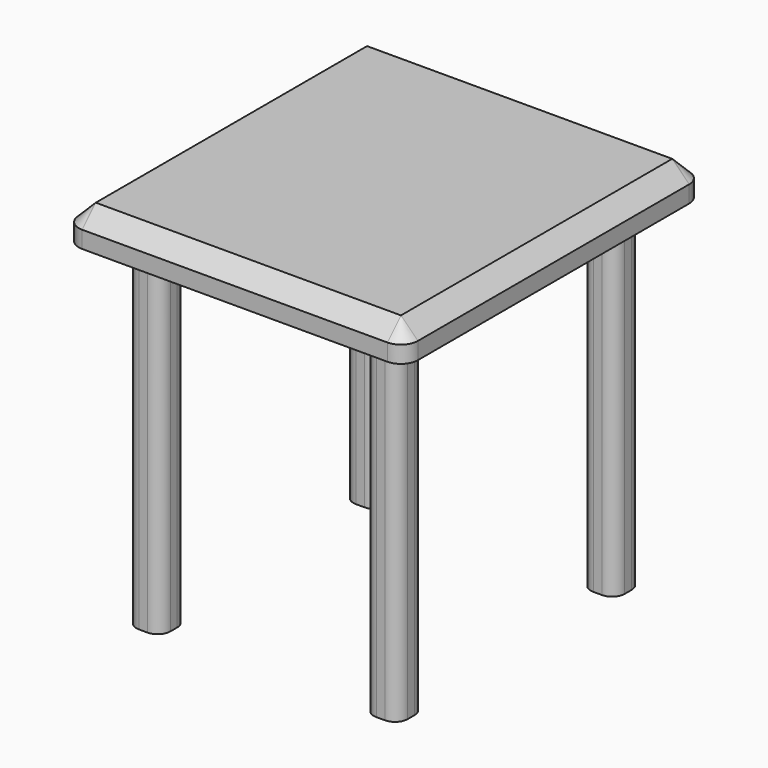
from build123d import *

# Parameters (mm, degrees)
F1_DEPTH = 40
F3_DEPTH = 400
F4_SIZE  = 19.99999


# Not quite as in the source:
# - a fillet or chamfer is up to 0.001 mm smaller than in the source, because OpenCascade refuses the exact size


with BuildPart() as f1:
    # F0 (on Top) → F1 (new body)
    with BuildSketch(Plane.XY):
        with BuildLine():
            Line((182.8182994574, 235.7496355578), (-177.1817005426, 235.7496355578))
            ThreePointArc((-177.1817005426, 235.7496355578), (-191.3238361663, 229.8917711815), (-197.1817005426, 215.7496355578))
            Line((-197.1817005426, 215.7496355578), (-197.1817005426, -184.2503644422))
            ThreePointArc((-197.1817005426, -184.2503644422), (-191.3238361663, -198.3925000659), (-177.1817005426, -204.2503644422))
            Line((-177.1817005426, -204.2503644422), (182.8182994574, -204.2503644422))
            ThreePointArc((182.8182994574, -204.2503644422), (196.9604350812, -198.3925000659), (202.8182994574, -184.2503644422))
            Line((202.8182994574, -184.2503644422), (202.8182994574, 215.7496355578))
            ThreePointArc((202.8182994574, 215.7496355578), (196.9604350812, 229.8917711815), (182.8182994574, 235.7496355578))
        make_face()
    extrude(amount=F1_DEPTH)

    # F2 (on face) → F3 (join)
    with BuildSketch(Plane(origin=(0, 0, 0), x_dir=(1, 0, 0), z_dir=(0, 0, -1))):
        with BuildLine():
            Line((-155.6743295648, -195.7496355578), (-132.1817005426, -195.7496355578))
            ThreePointArc((-132.1817005426, -195.7496355578), (-121.5750988248, -191.3562372756), (-117.1817005426, -180.7496355578))
            Line((-117.1817005426, -180.7496355578), (-117.1817005426, -170.7496355578))
            ThreePointArc((-117.1817005426, -170.7496355578), (-121.5750988248, -160.14303384), (-132.1817005426, -155.7496355578))
            Line((-132.1817005426, -155.7496355578), (-142.1817005426, -155.7496355578))
            ThreePointArc((-142.1817005426, -155.7496355578), (-152.7883022604, -160.14303384), (-157.1817005426, -170.7496355578))
            Line((-157.1817005426, -170.7496355578), (-157.1817005426, -194.2422645801))
            ThreePointArc((-157.1817005426, -194.2422645801), (-156.740201805, -195.3081368202), (-155.6743295648, -195.7496355578))
        make_face()
        with BuildLine():
            Line((124.3256704352, -195.7496355578), (147.8182994574, -195.7496355578))
            ThreePointArc((147.8182994574, -195.7496355578), (158.4249011752, -191.3562372756), (162.8182994574, -180.7496355578))
            Line((162.8182994574, -180.7496355578), (162.8182994574, -170.7496355578))
            ThreePointArc((162.8182994574, -170.7496355578), (158.4249011752, -160.14303384), (147.8182994574, -155.7496355578))
            Line((147.8182994574, -155.7496355578), (137.8182994574, -155.7496355578))
            ThreePointArc((137.8182994574, -155.7496355578), (127.2116977396, -160.14303384), (122.8182994574, -170.7496355578))
            Line((122.8182994574, -170.7496355578), (122.8182994574, -194.2422645801))
            ThreePointArc((122.8182994574, -194.2422645801), (123.259798195, -195.3081368202), (124.3256704352, -195.7496355578))
        make_face()
        with BuildLine():
            Line((124.3256704352, 124.2503644422), (147.8182994574, 124.2503644422))
            ThreePointArc((147.8182994574, 124.2503644422), (158.4249011752, 128.6437627244), (162.8182994574, 139.2503644422))
            Line((162.8182994574, 139.2503644422), (162.8182994574, 149.2503644422))
            ThreePointArc((162.8182994574, 149.2503644422), (158.4249011752, 159.85696616), (147.8182994574, 164.2503644422))
            Line((147.8182994574, 164.2503644422), (137.8182994574, 164.2503644422))
            ThreePointArc((137.8182994574, 164.2503644422), (127.2116977396, 159.85696616), (122.8182994574, 149.2503644422))
            Line((122.8182994574, 149.2503644422), (122.8182994574, 125.7577354199))
            ThreePointArc((122.8182994574, 125.7577354199), (123.259798195, 124.6918631798), (124.3256704352, 124.2503644422))
        make_face()
        with BuildLine():
            Line((-155.6743295648, 124.2503644422), (-132.1817005426, 124.2503644422))
            ThreePointArc((-132.1817005426, 124.2503644422), (-121.5750988248, 128.6437627244), (-117.1817005426, 139.2503644422))
            Line((-117.1817005426, 139.2503644422), (-117.1817005426, 149.2503644422))
            ThreePointArc((-117.1817005426, 149.2503644422), (-121.5750988248, 159.85696616), (-132.1817005426, 164.2503644422))
            Line((-132.1817005426, 164.2503644422), (-142.1817005426, 164.2503644422))
            ThreePointArc((-142.1817005426, 164.2503644422), (-152.7883022604, 159.85696616), (-157.1817005426, 149.2503644422))
            Line((-157.1817005426, 149.2503644422), (-157.1817005426, 125.7577354199))
            ThreePointArc((-157.1817005426, 125.7577354199), (-156.740201805, 124.6918631798), (-155.6743295648, 124.2503644422))
        make_face()
    extrude(amount=F3_DEPTH)

    # F4 (size 20 in the source; OpenCascade refuses exactly that, so slightly less here)
    f4_edges = [f1.edges().sort_by_distance(p)[0] for p in [
        (2.818299, 235.749636, 40),
        (-191.323836, 229.891771, 40),
        (-197.181701, 15.749636, 40),
        (-191.323836, -198.3925, 40),
        (2.818299, -204.250364, 40),
        (196.960435, -198.3925, 40),
        (202.818299, 15.749636, 40),
        (196.960435, 229.891771, 40),
    ]]
    chamfer(f4_edges, length=F4_SIZE)


solid = f1.part
